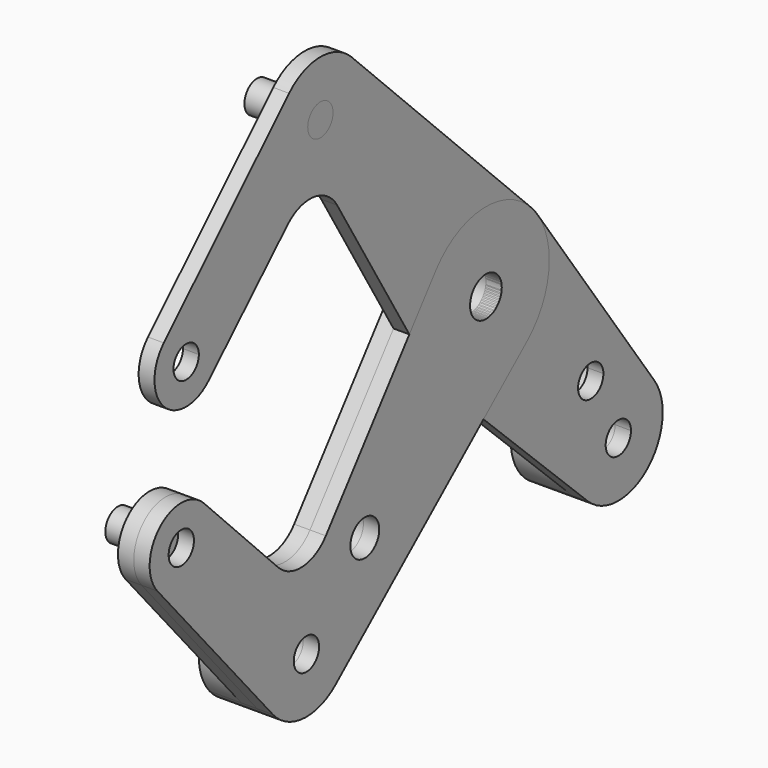
from build123d import *

# Parameters (mm, degrees)
F2_DEPTH = 3.175
F1_R     = 3.175
F1_R_2   = 3.6122259131
F1_R_3   = 3.9751
F3_DEPTH = 3.175
F4_R     = 3.175
F6_DEPTH = 9.525
F7_DEPTH = 9.525


with BuildPart() as f2:
    # F0 (on Right) → F2 (new body)
    with BuildSketch(Plane.YZ):
        with BuildLine():
            ThreePointArc((-69.1325679357, 24.2095168657), (-74.8432263912, 26.9547565738), (-80.7436939481, 24.6455481248))
            ThreePointArc((-80.7436939481, 24.6455481248), (-80.7830017069, 13.4395898025), (-69.5772444737, 13.3617961545))
            ThreePointArc((-69.5772444737, 13.3617961545), (-67.8210190346, 15.9535753265), (-67.2035924475, 19.022847468))
            ThreePointArc((-67.2035924475, 19.022847468), (-67.7014496617, 21.7897268417), (-69.1325679357, 24.2095168657))
        make_face()
        with BuildLine():
            ThreePointArc((-71.9660924475, 19.022847468), (-78.1169495619, 17.9160957186), (-72.7376826428, 21.0975152271))
            ThreePointArc((-72.7376826428, 21.0975152271), (-72.1652353332, 20.1295992175), (-71.9660924475, 19.022847468))
        make_face(mode=Mode.SUBTRACT)
        with BuildLine():
            Line((-49.336997282, 55.9399770143), (-80.7436939481, 24.6455481248))
            ThreePointArc((-80.7436939481, 24.6455481248), (-74.8432263912, 26.9547565738), (-69.1325679357, 24.2095168657))
            Line((-69.1325679357, 24.2095168657), (-49.9052894977, 40.8068589381))
            ThreePointArc((-49.9052894977, 40.8068589381), (-52.5980279292, 48.4852085737), (-49.336997282, 55.9399770143))
        make_face()
        with BuildLine():
            ThreePointArc((-67.2035924475, 19.022847468), (-67.8210190346, 15.9535753265), (-69.5772444737, 13.3617961545))
            Line((-69.5772444737, 13.3617961545), (-49.7042712662, 32.8935395696))
            ThreePointArc((-49.7042712662, 32.8935395696), (-43.1269205627, 35.1099036595), (-37.3152516644, 31.3153922718))
            Line((-37.3152516644, 31.3153922718), (-13.6107617236, -8.1708500356))
            ThreePointArc((-13.6107617236, -8.1708500356), (-15.6747276382, 2.5136703181), (-10.3733387953, 12.0170490237))
            Line((-10.3733387953, 12.0170490237), (-34.2320180244, 39.6562617782))
            ThreePointArc((-34.2320180244, 39.6562617782), (-42.3069502353, 36.9855195527), (-49.9052894977, 40.8068589381))
            Line((-49.9052894977, 40.8068589381), (-69.1325679357, 24.2095168657))
            ThreePointArc((-69.1325679357, 24.2095168657), (-67.7014496617, 21.7897268417), (-67.2035924475, 19.022847468))
        make_face()
        with BuildLine():
            ThreePointArc((-33.6497130803, 55.9399770143), (-41.4933551811, 59.1806960948), (-49.336997282, 55.9399770143))
            ThreePointArc((-49.336997282, 55.9399770143), (-52.5980279292, 48.4852085737), (-49.9052894977, 40.8068589381))
            Line((-49.9052894977, 40.8068589381), (-43.8967649859, 45.9935283358))
            ThreePointArc((-43.8967649859, 45.9935283358), (-42.6001069306, 51.0440532092), (-38.3183551811, 48.0681960948))
            ThreePointArc((-38.3183551811, 48.0681960948), (-38.6065147686, 46.7465390166), (-39.4186874221, 45.6647862901))
            Line((-39.4186874221, 45.6647862901), (-34.2320180244, 39.6562617782))
            ThreePointArc((-34.2320180244, 39.6562617782), (-31.3894137372, 43.442396321), (-30.3808551811, 48.0681960948))
            ThreePointArc((-30.3808551811, 48.0681960948), (-31.2305551467, 52.3299553211), (-33.6497130803, 55.9399770143))
        make_face()
        with BuildLine():
            Line((11.2052030012, 11.2454013135), (-33.6497130803, 55.9399770143))
            ThreePointArc((-33.6497130803, 55.9399770143), (-31.2305551467, 52.3299553211), (-30.3808551811, 48.0681960948))
            ThreePointArc((-30.3808551811, 48.0681960948), (-31.3894137372, 43.442396321), (-34.2320180244, 39.6562617782))
            Line((-34.2320180244, 39.6562617782), (-10.3733387953, 12.0170490237))
            ThreePointArc((-10.3733387953, 12.0170490237), (0.5673266796, 15.8648594522), (11.2052030012, 11.2454013135))
        make_face()
        with BuildLine():
            ThreePointArc((12.9366236895, 9.2010538807), (12.114115242, 10.2598166116), (11.2052030012, 11.2454013135))
            ThreePointArc((11.2052030012, 11.2454013135), (0.5673266796, 15.8648594522), (-10.3733387953, 12.0170490237))
            Line((-10.3733387953, 12.0170490237), (-2.5974840343, 3.0090690755))
            ThreePointArc((-2.5974840343, 3.0090690755), (1.654714662, 3.6143241965), (3.9751, 0))
            ThreePointArc((3.9751, 0), (3.6143241965, -1.654714662), (2.5974840343, -3.0090690755))
            Line((2.5974840343, -3.0090690755), (10.3733387953, -12.0170490237))
            ThreePointArc((10.3733387953, -12.0170490237), (14.4342020627, -6.6082853913), (15.875, 0))
            ThreePointArc((15.875, 0), (15.1225746166, 4.8294266704), (12.9366236895, 9.2010538807))
        make_face()
        with BuildLine():
            ThreePointArc((-10.3733387953, 12.0170490237), (-15.6747276382, 2.5136703181), (-13.6107617236, -8.1708500356))
            ThreePointArc((-13.6107617236, -8.1708500356), (-12.4102582236, -9.899551294), (-10.9916226654, -11.4542505727))
            ThreePointArc((-10.9916226654, -11.4542505727), (-0.4180361948, -15.8694949743), (10.3733387953, -12.0170490237))
            Line((10.3733387953, -12.0170490237), (2.5974840343, -3.0090690755))
            ThreePointArc((2.5974840343, -3.0090690755), (-3.0090690755, -2.5974840343), (-2.5974840343, 3.0090690755))
            Line((-2.5974840343, 3.0090690755), (-10.3733387953, 12.0170490237))
        make_face()
        with BuildLine():
            Line((42.2503207276, -32.0138191594), (12.9366236895, 9.2010538807))
            ThreePointArc((12.9366236895, 9.2010538807), (15.1225746166, 4.8294266704), (15.875, 0))
            ThreePointArc((15.875, 0), (14.4342020627, -6.6082853913), (10.3733387953, -12.0170490237))
            Line((10.3733387953, -12.0170490237), (23.8669779002, -27.6488263938))
            Line((23.8669779002, -27.6488263938), (25.9333469882, -30.0426225593))
            ThreePointArc((25.9333469882, -30.0426225593), (34.5274562997, -27.4222690518), (42.2503207276, -32.0138191594))
        make_face()
        with BuildLine():
            ThreePointArc((29.4453877049, -25.5741586347), (27.3771394544, -28.550015749), (23.8669779002, -27.6488263938))
            ThreePointArc((23.8669779002, -27.6488263938), (25.1636359555, -22.5983015203), (29.4453877049, -25.5741586347))
        make_face(mode=Mode.SUBTRACT)
        with BuildLine():
            ThreePointArc((10.3733387953, -12.0170490237), (-0.4180361948, -15.8694949743), (-10.9916226654, -11.4542505727))
            Line((-10.9916226654, -11.4542505727), (25.5005482791, -46.4725322767))
            ThreePointArc((25.5005482791, -46.4725322767), (22.0860376629, -38.1619315395), (25.9333469882, -30.0426225593))
            Line((25.9333469882, -30.0426225593), (23.8669779002, -27.6488263938))
            Line((23.8669779002, -27.6488263938), (10.3733387953, -12.0170490237))
        make_face()
        with BuildLine():
            ThreePointArc((44.3071841449, -38.4545568759), (43.7804863765, -35.0739582066), (42.2503207276, -32.0138191594))
            ThreePointArc((42.2503207276, -32.0138191594), (34.5274562997, -27.4222690518), (25.9333469882, -30.0426225593))
            ThreePointArc((25.9333469882, -30.0426225593), (22.0860376629, -38.1619315395), (25.5005482791, -46.4725322767))
            ThreePointArc((25.5005482791, -46.4725322767), (37.5528128398, -48.6768056759), (44.3071841449, -38.4545568759))
        make_face()
        with BuildLine():
            ThreePointArc((36.3696841449, -38.4545568759), (31.8730270667, -41.3413972884), (31.1200163859, -36.0511470711))
            ThreePointArc((31.1200163859, -36.0511470711), (34.5163412232, -35.5677164633), (36.3696841449, -38.4545568759))
        make_face(mode=Mode.SUBTRACT)
        with BuildLine():
            Line((-43.8967649859, 45.9935283358), (-49.9052894977, 40.8068589381))
            ThreePointArc((-49.9052894977, 40.8068589381), (-42.3069502353, 36.9855195527), (-34.2320180244, 39.6562617782))
            Line((-34.2320180244, 39.6562617782), (-39.4186874221, 45.6647862901))
            ThreePointArc((-39.4186874221, 45.6647862901), (-41.7258109109, 44.9017170828), (-43.8967649859, 45.9935283358))
        make_face()
    extrude(amount=F2_DEPTH)

    # F0 (on Right) + F4 (on face) → F6 (join, through all)
    with BuildSketch(Plane.YZ):
        with BuildLine():
            ThreePointArc((-38.3183551811, 48.0681960948), (-42.6001069306, 51.0440532092), (-43.8967649859, 45.9935283358))
            Line((-43.8967649859, 45.9935283358), (-41.4933551811, 48.0681960948))
            Line((-41.4933551811, 48.0681960948), (-39.4186874221, 45.6647862901))
            ThreePointArc((-39.4186874221, 45.6647862901), (-38.6065147686, 46.7465390166), (-38.3183551811, 48.0681960948))
        make_face()
        with BuildLine():
            Line((-41.4933551811, 48.0681960948), (-43.8967649859, 45.9935283358))
            ThreePointArc((-43.8967649859, 45.9935283358), (-41.7258109109, 44.9017170828), (-39.4186874221, 45.6647862901))
            Line((-39.4186874221, 45.6647862901), (-41.4933551811, 48.0681960948))
        make_face()
        with BuildLine():
            ThreePointArc((44.3071841449, -38.4545568759), (43.7804863765, -35.0739582066), (42.2503207276, -32.0138191594))
            ThreePointArc((42.2503207276, -32.0138191594), (34.5274562997, -27.4222690518), (25.9333469882, -30.0426225593))
            ThreePointArc((25.9333469882, -30.0426225593), (22.0860376629, -38.1619315395), (25.5005482791, -46.4725322767))
            ThreePointArc((25.5005482791, -46.4725322767), (37.5528128398, -48.6768056759), (44.3071841449, -38.4545568759))
        make_face()
        with BuildLine():
            ThreePointArc((36.3696841449, -38.4545568759), (31.8730270667, -41.3413972884), (31.1200163859, -36.0511470711))
            ThreePointArc((31.1200163859, -36.0511470711), (34.5163412232, -35.5677164633), (36.3696841449, -38.4545568759))
        make_face(mode=Mode.SUBTRACT)
    with BuildSketch(Plane.YZ.offset(3.175)):
        with Locations((-41.4933551811, 48.0681960948)):
            Circle(F4_R)
    extrude(amount=-F6_DEPTH)


with BuildPart() as f2b:
    # F1 (on Right) → F2, piece 2 (new body)
    with BuildSketch(Plane.YZ):
        with BuildLine():
            ThreePointArc((-82.370280796, -18.4955128706), (-73.5944347637, -20.7507160795), (-68.4226920805, -13.3106560855))
            ThreePointArc((-68.4226920805, -13.3106560855), (-69.0157041836, -10.3002734217), (-70.7061324036, -7.7397032567))
            ThreePointArc((-70.7061324036, -7.7397032567), (-81.7410423183, -7.4753877139), (-82.370280796, -18.4955128706))
        make_face()
        with Locations((-76.3601920805, -13.3106560855)):
            Circle(F1_R, mode=Mode.SUBTRACT)
        with BuildLine():
            ThreePointArc((-70.7061324036, -7.7397032567), (-69.0157041836, -10.3002734217), (-68.4226920805, -13.3106560855))
            ThreePointArc((-68.4226920805, -13.3106560855), (-73.5944347637, -20.7507160795), (-82.370280796, -18.4955128706))
            Line((-82.370280796, -18.4955128706), (-53.4092469001, -52.0660414735))
            ThreePointArc((-53.4092469001, -52.0660414735), (-52.5499819735, -36.6579010449), (-37.1209762262, -36.9659746289))
            ThreePointArc((-37.1209762262, -36.9659746289), (-34.7240684945, -40.5654143272), (-33.8826226985, -44.8072419744))
            ThreePointArc((-33.8826226985, -44.8072419744), (-34.9001805283, -49.4526481816), (-37.7665010031, -53.2473062298))
            Line((-37.7665010031, -53.2473062298), (10.3266024219, -12.0572346506))
            ThreePointArc((10.3266024219, -12.0572346506), (-10.9422363509, -11.5014385466), (-12.5565456786, 9.7133303054))
            Line((-12.5565456786, 9.7133303054), (-40.1280920851, -25.9287585557))
            ThreePointArc((-40.1280920851, -25.9287585557), (-45.9413494341, -29.0003165232), (-52.0795163333, -26.644189092))
            Line((-52.0795163333, -26.644189092), (-70.7061324036, -7.7397032567))
        make_face()
        with Locations((-30.3627087969, -30.2359268843)):
            Circle(F1_R_2, mode=Mode.SUBTRACT)
        with BuildLine():
            ThreePointArc((-37.1209762262, -36.9659746289), (-52.5499819735, -36.6579010449), (-53.4092469001, -52.0660414735))
            ThreePointArc((-53.4092469001, -52.0660414735), (-45.8319026302, -55.8881920959), (-37.7665010031, -53.2473062298))
            Line((-37.7665010031, -53.2473062298), (-37.1209762262, -36.9659746289))
        make_face()
        with Locations((-44.9951226985, -44.8072419744)):
            Circle(F1_R, mode=Mode.SUBTRACT)
        with BuildLine():
            ThreePointArc((-33.8826226985, -44.8072419744), (-34.7240684945, -40.5654143272), (-37.1209762262, -36.9659746289))
            Line((-37.1209762262, -36.9659746289), (-37.7665010031, -53.2473062298))
            ThreePointArc((-37.7665010031, -53.2473062298), (-34.9001805283, -49.4526481816), (-33.8826226985, -44.8072419744))
        make_face()
        with BuildLine():
            ThreePointArc((15.875, 0), (5.13227349, 15.0224962581), (-12.5565456786, 9.7133303054))
            ThreePointArc((-12.5565456786, 9.7133303054), (-10.9422363509, -11.5014385466), (10.3266024219, -12.0572346506))
            ThreePointArc((10.3266024219, -12.0572346506), (14.4213459574, -6.6362945818), (15.875, 0))
        make_face()
        Circle(F1_R_3, mode=Mode.SUBTRACT)
    extrude(amount=F2_DEPTH)


with BuildPart() as f3:
    # F1 (on Right) → F3 (new body)
    with BuildSketch(Plane.YZ):
        with BuildLine():
            ThreePointArc((-82.370280796, -18.4955128706), (-73.5944347637, -20.7507160795), (-68.4226920805, -13.3106560855))
            ThreePointArc((-68.4226920805, -13.3106560855), (-69.0157041836, -10.3002734217), (-70.7061324036, -7.7397032567))
            ThreePointArc((-70.7061324036, -7.7397032567), (-81.7410423183, -7.4753877139), (-82.370280796, -18.4955128706))
        make_face()
        with Locations((-76.3601920805, -13.3106560855)):
            Circle(F1_R, mode=Mode.SUBTRACT)
        with BuildLine():
            ThreePointArc((-70.7061324036, -7.7397032567), (-69.0157041836, -10.3002734217), (-68.4226920805, -13.3106560855))
            ThreePointArc((-68.4226920805, -13.3106560855), (-73.5944347637, -20.7507160795), (-82.370280796, -18.4955128706))
            Line((-82.370280796, -18.4955128706), (-53.4092469001, -52.0660414735))
            ThreePointArc((-53.4092469001, -52.0660414735), (-52.5499819735, -36.6579010449), (-37.1209762262, -36.9659746289))
            ThreePointArc((-37.1209762262, -36.9659746289), (-34.7240684945, -40.5654143272), (-33.8826226985, -44.8072419744))
            ThreePointArc((-33.8826226985, -44.8072419744), (-34.9001805283, -49.4526481816), (-37.7665010031, -53.2473062298))
            Line((-37.7665010031, -53.2473062298), (10.3266024219, -12.0572346506))
            ThreePointArc((10.3266024219, -12.0572346506), (-10.9422363509, -11.5014385466), (-12.5565456786, 9.7133303054))
            Line((-12.5565456786, 9.7133303054), (-40.1280920851, -25.9287585557))
            ThreePointArc((-40.1280920851, -25.9287585557), (-45.9413494341, -29.0003165232), (-52.0795163333, -26.644189092))
            Line((-52.0795163333, -26.644189092), (-70.7061324036, -7.7397032567))
        make_face()
        with Locations((-30.3627087969, -30.2359268843)):
            Circle(F1_R_2, mode=Mode.SUBTRACT)
        with BuildLine():
            ThreePointArc((-37.1209762262, -36.9659746289), (-52.5499819735, -36.6579010449), (-53.4092469001, -52.0660414735))
            ThreePointArc((-53.4092469001, -52.0660414735), (-45.8319026302, -55.8881920959), (-37.7665010031, -53.2473062298))
            Line((-37.7665010031, -53.2473062298), (-37.1209762262, -36.9659746289))
        make_face()
        with Locations((-44.9951226985, -44.8072419744)):
            Circle(F1_R, mode=Mode.SUBTRACT)
        with BuildLine():
            ThreePointArc((-33.8826226985, -44.8072419744), (-34.7240684945, -40.5654143272), (-37.1209762262, -36.9659746289))
            Line((-37.1209762262, -36.9659746289), (-37.7665010031, -53.2473062298))
            ThreePointArc((-37.7665010031, -53.2473062298), (-34.9001805283, -49.4526481816), (-33.8826226985, -44.8072419744))
        make_face()
        with BuildLine():
            ThreePointArc((15.875, 0), (5.13227349, 15.0224962581), (-12.5565456786, 9.7133303054))
            ThreePointArc((-12.5565456786, 9.7133303054), (-10.9422363509, -11.5014385466), (10.3266024219, -12.0572346506))
            ThreePointArc((10.3266024219, -12.0572346506), (14.4213459574, -6.6362945818), (15.875, 0))
        make_face()
        Circle(F1_R_3, mode=Mode.SUBTRACT)
    extrude(amount=-F3_DEPTH)


with BuildPart() as f6:
    # F1 (on Right) → F6, piece 2 (new body, through all)
    with BuildSketch(Plane.YZ):
        with Locations((-76.3601920805, -13.3106560855)):
            Circle(F1_R)
    extrude(amount=-F6_DEPTH)


with BuildPart() as f7:
    # F1 (on Right) → F7 (new body, through all)
    with BuildSketch(Plane.YZ):
        with BuildLine():
            ThreePointArc((-37.1209762262, -36.9659746289), (-52.5499819735, -36.6579010449), (-53.4092469001, -52.0660414735))
            ThreePointArc((-53.4092469001, -52.0660414735), (-45.8319026302, -55.8881920959), (-37.7665010031, -53.2473062298))
            Line((-37.7665010031, -53.2473062298), (-37.1209762262, -36.9659746289))
        make_face()
        with Locations((-44.9951226985, -44.8072419744)):
            Circle(F1_R, mode=Mode.SUBTRACT)
    extrude(amount=-F7_DEPTH)


solid = Compound([f2.part, f2b.part, f3.part, f6.part, f7.part])
